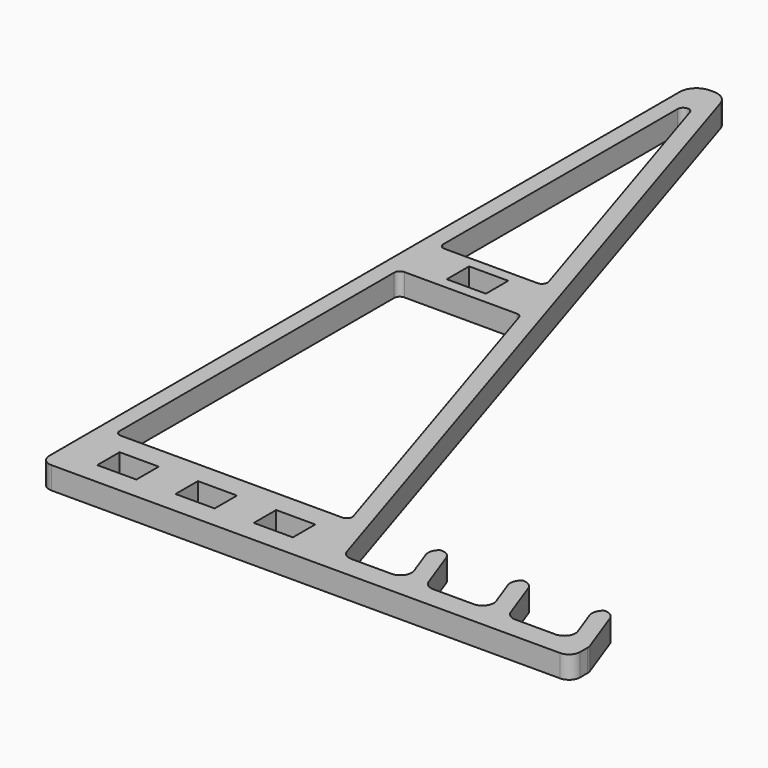
from build123d import *

# Parameters (mm, degrees)
F0_W        = 7
F0_H        = 5
F1_DEPTH    = 4
F2_T1_DEPTH = 4
F2_T3_DEPTH = 14
F2_T5_DEPTH = 5.7632698071


# Not quite as in the source:
# - a fillet or chamfer that OpenCascade refuses, or shapes differently, is made with other operations: its cross-section is extruded or revolved along the edge and cut away or added


with BuildPart() as f1:
    # F0 (on Top) → F1 (new body)
    with BuildSketch(Plane.XY):
        with BuildLine():
            Line((-51, -4), (44, -4))
            Line((44, -4), (44, 0))
            Line((44, 0), (40.8074666826, 0))
            Line((40.8074666826, 0), (29.3850666349, 0))
            Line((29.3850666349, 0), (26.1925333174, 0))
            Line((26.1925333174, 0), (14.6925333174, 0))
            Line((14.6925333174, 0), (11.5, 0))
            Line((11.5, 0), (0, 0))
            Line((0, 0), (-44.4302483166, 139.9080159757))
            ThreePointArc((-44.4302483166, 139.9080159757), (-45.5180993372, 141.4211616971), (-47.2895326655, 142))
            Line((-47.2895326655, 142), (-48, 142))
            ThreePointArc((-48, 142), (-50.1213203436, 141.1213203436), (-51, 139))
            Line((-51, 139), (-51, -4))
        make_face()
        with Locations((-40.5, 2.5)):
            Rectangle(F0_W, F0_H, mode=Mode.SUBTRACT)
        with Locations((-26.5, 2.5)):
            Rectangle(F0_W, F0_H, mode=Mode.SUBTRACT)
        with Locations((-12.5, 2.5)):
            Rectangle(F0_W, F0_H, mode=Mode.SUBTRACT)
        with BuildLine():
            Line((-7.3725300405, 9), (-47, 9))
            ThreePointArc((-47, 9), (-47.7071067812, 9.2928932188), (-48, 10))
            Line((-48, 10), (-48, 71.4074290533))
            ThreePointArc((-48, 71.4074290533), (-47.7071067812, 72.1145358345), (-47, 72.4074290533))
            Line((-47, 72.4074290533), (-26.8735379155, 72.4074290533))
            ThreePointArc((-26.8735379155, 72.4074290533), (-26.2830601394, 72.2144829523), (-25.9204431326, 71.7101010452))
            Line((-25.9204431326, 71.7101010452), (-6.4194352575, 10.3026719919))
            ThreePointArc((-6.4194352575, 10.3026719919), (-6.5654761415, 9.4095222239), (-7.3725300405, 9))
        make_face(mode=Mode.SUBTRACT)
        with Locations((-37.5, 76.9074290533)):
            Rectangle(F0_W, F0_H, mode=Mode.SUBTRACT)
        with BuildLine():
            ThreePointArc((-48, 134.7843734895), (-47.1531424452, 135.7725776139), (-46.046905217, 135.0870454814))
            Line((-46.046905217, 135.0870454814), (-29.4136863758, 82.7101010452))
            ThreePointArc((-29.4136863758, 82.7101010452), (-29.5597272597, 81.8169512772), (-30.3667811588, 81.4074290533))
            Line((-30.3667811588, 81.4074290533), (-47, 81.4074290533))
            ThreePointArc((-47, 81.4074290533), (-47.7071067812, 81.7003222721), (-48, 82.4074290533))
            Line((-48, 82.4074290533), (-48, 134.7843734895))
        make_face(mode=Mode.SUBTRACT)
        Polygon((40.8074666826, 0), (44, 0), (40.2063431117, 10.4229866378), (37.3872652493, 9.3969262079), align=None)
        Polygon((26.1925333174, 0), (29.3850666349, 0), (25.5914097465, 10.4229866378), (22.7723318842, 9.3969262079), align=None)
        Polygon((11.5, 0), (14.6925333174, 0), (10.8988764291, 10.4229866378), (8.0797985667, 9.3969262079), align=None)
    extrude(amount=F1_DEPTH)

    # F2: fillet of radius 2 on 15 edges, made by hand

    # F2_s2 → F2_t1 (join)
    with BuildSketch(Plane.XY):
        with BuildLine():
            ThreePointArc((39.8305559107, 2.6840402867), (39.5894747577, 0.8528471273), (37.9511706691, 0))
            Line((37.9511706691, 0), (40.8074666826, 0))
            Line((40.8074666826, 0), (39.8305559107, 2.6840402867))
        make_face()
        with BuildLine():
            ThreePointArc((16.0929483938, 0), (14.9457955211, 0.3616959114), (14.2135631523, 1.3159597133))
            Line((14.2135631523, 1.3159597133), (14.6925333174, 0))
            Line((14.6925333174, 0), (16.0929483938, 0))
        make_face()
        with BuildLine():
            ThreePointArc((10.5230892281, 2.6840402867), (10.2820080751, 0.8528471273), (8.6437039865, 0))
            Line((8.6437039865, 0), (11.5, 0))
            Line((11.5, 0), (10.5230892281, 2.6840402867))
        make_face()
        with BuildLine():
            ThreePointArc((1.4632920473, 0), (0.2823364951, 0.3858922019), (-0.4428975187, 1.3946560162))
            Line((-0.4428975187, 1.3946560162), (0, 0))
            Line((0, 0), (1.4632920473, 0))
        make_face()
        with BuildLine():
            ThreePointArc((25.2156225455, 2.6840402867), (24.9745413925, 0.8528471273), (23.3362373039, 0))
            Line((23.3362373039, 0), (26.1925333174, 0))
            Line((26.1925333174, 0), (25.2156225455, 2.6840402867))
        make_face()
        with BuildLine():
            ThreePointArc((30.7854817113, 0), (29.6383288386, 0.3616959114), (28.9060964697, 1.3159597133))
            Line((28.9060964697, 1.3159597133), (29.3850666349, 0))
            Line((29.3850666349, 0), (30.7854817113, 0))
        make_face()
    extrude(amount=F2_T1_DEPTH)

    # F2_s4 → F2_t3 (cut)
    with BuildSketch(Plane.XY.offset(-5)):
        with BuildLine():
            ThreePointArc((-51, -2), (-50.4142135624, -3.4142135624), (-49, -4))
            Line((-49, -4), (-51, -4))
            Line((-51, -4), (-51, -2))
        make_face()
        with BuildLine():
            ThreePointArc((42, -4), (43.4142135624, -3.4142135624), (44, -2))
            Line((44, -2), (44, -4))
            Line((44, -4), (42, -4))
        make_face()
        with BuildLine():
            ThreePointArc((40.8903833983, 8.5436013963), (39.8562346802, 9.6721766837), (38.3269578701, 9.7389463512))
            Line((38.3269578701, 9.7389463512), (40.2063431117, 10.4229866378))
            Line((40.2063431117, 10.4229866378), (40.8903833983, 8.5436013963))
        make_face()
        with BuildLine():
            ThreePointArc((39.2666504909, 10.0809664945), (38.1380752035, 9.0468177764), (38.071305536, 7.5175409663))
            Line((38.071305536, 7.5175409663), (37.3872652493, 9.3969262079))
            Line((37.3872652493, 9.3969262079), (39.2666504909, 10.0809664945))
        make_face()
        with BuildLine():
            ThreePointArc((11.5829167158, 8.5436013963), (10.5487679977, 9.6721766837), (9.0194911875, 9.7389463512))
            Line((9.0194911875, 9.7389463512), (10.8988764291, 10.4229866378))
            Line((10.8988764291, 10.4229866378), (11.5829167158, 8.5436013963))
        make_face()
        with BuildLine():
            ThreePointArc((9.9591838083, 10.0809664945), (8.8306085209, 9.0468177764), (8.7638388534, 7.5175409663))
            Line((8.7638388534, 7.5175409663), (8.0797985667, 9.3969262079))
            Line((8.0797985667, 9.3969262079), (9.9591838083, 10.0809664945))
        make_face()
        with BuildLine():
            ThreePointArc((24.6517171257, 10.0809664945), (23.5231418383, 9.0468177764), (23.4563721708, 7.5175409663))
            Line((23.4563721708, 7.5175409663), (22.7723318842, 9.3969262079))
            Line((22.7723318842, 9.3969262079), (24.6517171257, 10.0809664945))
        make_face()
        with BuildLine():
            ThreePointArc((26.2754500332, 8.5436013963), (25.2413013151, 9.6721766837), (23.712024505, 9.7389463512))
            Line((23.712024505, 9.7389463512), (25.5914097465, 10.4229866378))
            Line((25.5914097465, 10.4229866378), (26.2754500332, 8.5436013963))
        make_face()
    extrude(amount=F2_T3_DEPTH, mode=Mode.SUBTRACT)

    # F2_s6 → F2_t5 (cut)
    with BuildSketch(Plane.XY.offset(-0.8816349035)):
        with BuildLine():
            ThreePointArc((44, -0.3526539614), (43.969615506, -0.0053576061), (43.8793852416, 0.3313863252))
            Line((43.8793852416, 0.3313863252), (44, 0))
            Line((44, 0), (44, -0.3526539614))
        make_face()
    extrude(amount=F2_T5_DEPTH, mode=Mode.SUBTRACT)


solid = f1.part
